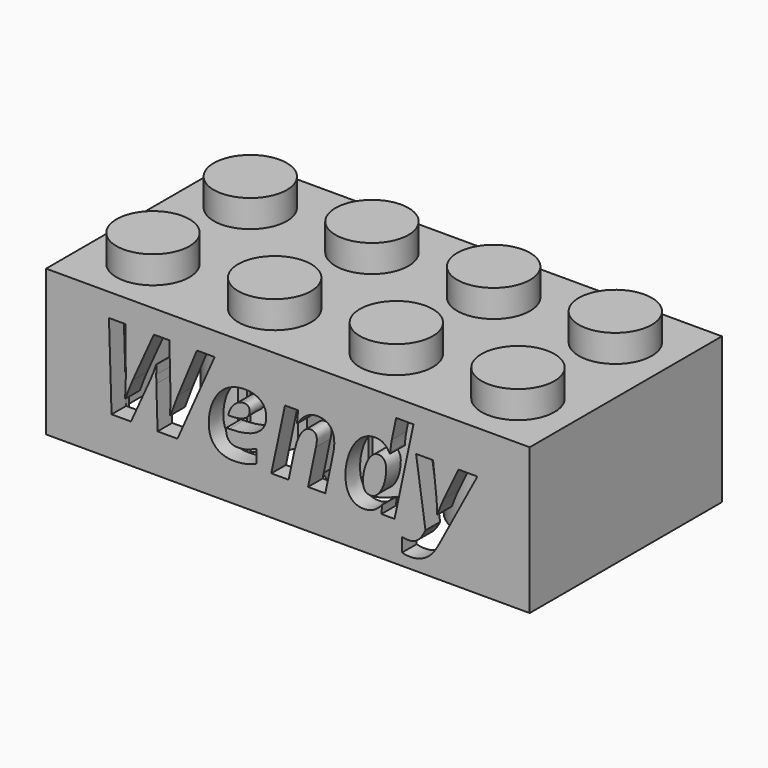
from build123d import *

# Parameters (mm, degrees)
F0_W          = 31.8
F0_H          = 15.8
F1_DEPTH      = 9.6
F2_W          = 29.4
F2_H          = 13.4
F3_DEPTH      = 8.4
F4_R          = 2.4
F5_DEPTH      = 1.8
F6_R          = 1.3
F7_DEPTH      = 1.2
F8_R          = 3.25
F8_R_2        = 2.4
F9_DEPTH      = 8.4
F10_W         = 0.6
F10_H         = 0.3
F11_DEPTH     = 8.6
F12_W         = 0.3
F12_H         = 0.6
F13_DEPTH     = 8.6
F14_W         = 0.6
F14_H         = 4
F15_DEPTH     = 6.4
F16_W         = 0.6
F16_H         = 4
F17_DEPTH     = 6.4
F18_TEXT_SIZE = 7.7383689738
F19_DEPTH     = 1.2


# Not quite as in the source:
# - Text() gives the source's letters only with a copy of the font that has no kerning and outlines rounded to 1/6400 em; it was checked with that copy


with BuildPart() as f1:
    # F0 (on Top) → F1 (new body)
    with BuildSketch(Plane.XY):
        Rectangle(F0_W, F0_H)
    extrude(amount=F1_DEPTH)

    # F2 (on face) → F3 (cut)
    with BuildSketch(Plane(origin=(0, 0, 0), x_dir=(1, 0, 0), z_dir=(0, 0, -1))):
        Rectangle(F2_W, F2_H)
    extrude(amount=-F3_DEPTH, mode=Mode.SUBTRACT)

    # F4 (on face) → F5 (join)
    with BuildSketch(Plane.XY.offset(9.6)):
        with Locations((-11.95, 3.95)):
            Circle(F4_R)
        with Locations((-11.95, -4.05)):
            Circle(F4_R)
        with Locations((-3.95, 3.95)):
            Circle(F4_R)
        with Locations((-3.95, -4.05)):
            Circle(F4_R)
        with Locations((4.05, 3.95)):
            Circle(F4_R)
        with Locations((4.05, -4.05)):
            Circle(F4_R)
        with Locations((12.05, 3.95)):
            Circle(F4_R)
        with Locations((12.05, -4.05)):
            Circle(F4_R)
    extrude(amount=F5_DEPTH)

    # F6 (on face) → F7 (cut)
    with BuildSketch(Plane(origin=(0, 0, 8.4), x_dir=(1, 0, 0), z_dir=(0, 0, -1))):
        with Locations((-11.95, 3.95)):
            Circle(F6_R)
        with Locations((-11.95, -4.05)):
            Circle(F6_R)
        with Locations((-3.95, 3.95)):
            Circle(F6_R)
        with Locations((-3.95, -4.05)):
            Circle(F6_R)
        with Locations((4.05, 3.95)):
            Circle(F6_R)
        with Locations((4.05, -4.05)):
            Circle(F6_R)
        with Locations((12.05, 3.95)):
            Circle(F6_R)
        with Locations((12.05, -4.05)):
            Circle(F6_R)
    extrude(amount=-F7_DEPTH, mode=Mode.SUBTRACT)

    # F8 (on face) → F9 (join, through all)
    with BuildSketch(Plane(origin=(0, 0, 8.4), x_dir=(1, 0, 0), z_dir=(0, 0, -1))):
        with Locations((-7.95, -0.05)):
            Circle(F8_R)
        with Locations((-7.95, -0.05)):
            Circle(F8_R_2, mode=Mode.SUBTRACT)
        with Locations((0.05, -0.05)):
            Circle(F8_R)
        with Locations((0.05, -0.05)):
            Circle(F8_R_2, mode=Mode.SUBTRACT)
        with Locations((8.05, -0.05)):
            Circle(F8_R)
        with Locations((8.05, -0.05)):
            Circle(F8_R_2, mode=Mode.SUBTRACT)
    extrude(amount=F9_DEPTH)

    # F10 (on face) → F11 (join)
    with BuildSketch(Plane(origin=(0, 0, 0), x_dir=(1, 0, 0), z_dir=(0, 0, -1))):
        with Locations((-11.95, 6.55)):
            Rectangle(F10_W, F10_H)
        with Locations((-11.95, -6.55)):
            Rectangle(F10_W, F10_H)
        with Locations((-3.95, 6.55)):
            Rectangle(F10_W, F10_H)
        with Locations((-3.95, -6.55)):
            Rectangle(F10_W, F10_H)
        with Locations((4.05, 6.55)):
            Rectangle(F10_W, F10_H)
        with Locations((4.05, -6.55)):
            Rectangle(F10_W, F10_H)
        with Locations((12.05, 6.55)):
            Rectangle(F10_W, F10_H)
        with Locations((12.05, -6.55)):
            Rectangle(F10_W, F10_H)
    extrude(amount=-F11_DEPTH)

    # F12 (on Top) → F13 (join)
    with BuildSketch(Plane.XY):
        with Locations((-14.55, -4.05)):
            Rectangle(F12_W, F12_H)
        with Locations((-14.55, 3.95)):
            Rectangle(F12_W, F12_H)
        with Locations((14.55, -4.05)):
            Rectangle(F12_W, F12_H)
        with Locations((14.55, 3.95)):
            Rectangle(F12_W, F12_H)
    extrude(amount=F13_DEPTH)

    # F14 (on face) → F15 (join)
    with BuildSketch(Plane(origin=(0, 0, 8.4), x_dir=(1, 0, 0), z_dir=(0, 0, -1))):
        with Locations((0, 5.0097692292)):
            Rectangle(F14_W, F14_H)
    extrude(amount=F15_DEPTH)

    # F16 (on face) → F17 (join)
    with BuildSketch(Plane(origin=(0, 0, 8.4), x_dir=(1, 0, 0), z_dir=(0, 0, -1))):
        with Locations((0, -5.0502038794)):
            Rectangle(F16_W, F16_H)
    extrude(amount=F17_DEPTH)

    # F18 (on face) → F19 (cut)
    with BuildSketch(Plane.XZ.offset(7.9)):
        with Locations((-12.4599831679, 2.562451642)):
            Text('Wendy', F18_TEXT_SIZE, font='Open Sans', font_style=FontStyle.BOLDITALIC, text_align=(TextAlign.LEFT, TextAlign.BOTTOM))
    extrude(amount=-F19_DEPTH, mode=Mode.SUBTRACT)


solid = f1.part
